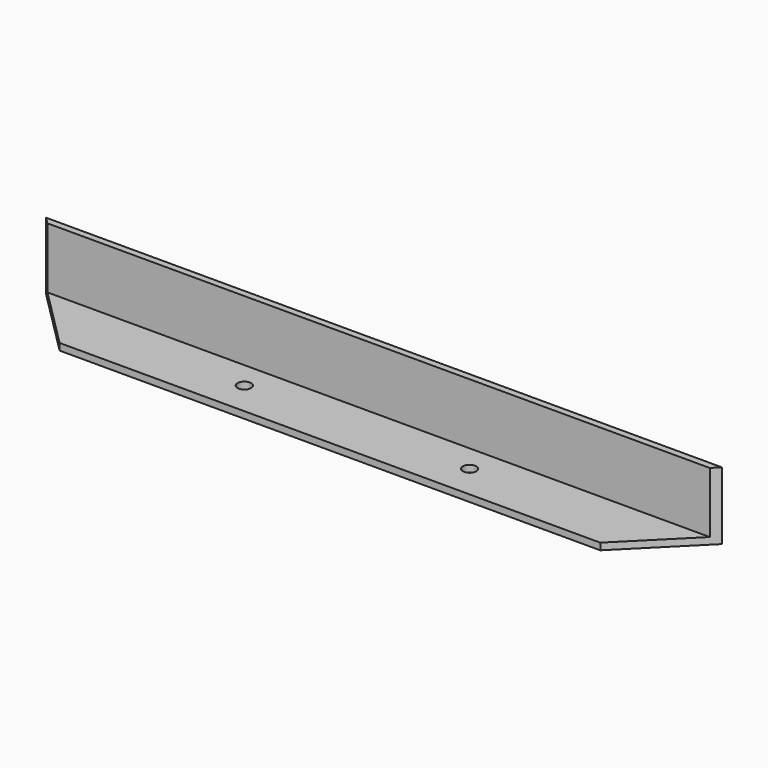
from build123d import *

# Parameters (mm, degrees)
F0_R     = 2.54
F1_DEPTH = 25.4
F2_T     = -2.54


# Not quite as in the source:
# - a feature names something its author has since deleted; it is built from what else it names


with BuildPart() as f1:
    # F0 (on Top) → F1 (new body)
    with BuildSketch(Plane.XY):
        Polygon((84.6666666667, 6.4318103081), (-169.3333333333, 6.4318103081), (-143.9333333333, -18.9681896919), (59.2666666667, -18.9681896919), align=None)
        with Locations((-84.6666666667, -6.2681896919)):
            Circle(F0_R, mode=Mode.SUBTRACT)
        with Locations((0, -6.2681896919)):
            Circle(F0_R, mode=Mode.SUBTRACT)
    extrude(amount=F1_DEPTH)

    # F2
    f2_openings = [f1.faces().sort_by_distance(p)[0] for p in [
        (71.966667, -6.26819, 12.7),
        (-156.633333, -6.26819, 12.7),
        (-42.333333, -18.96819, 12.7),
        (-42.333333, -5.794512, 25.4),
        (-87.206667, -6.26819, 12.7),
        (-2.54, -6.26819, 12.7),
    ]]
    offset(amount=F2_T, openings=f2_openings)


solid = f1.part
